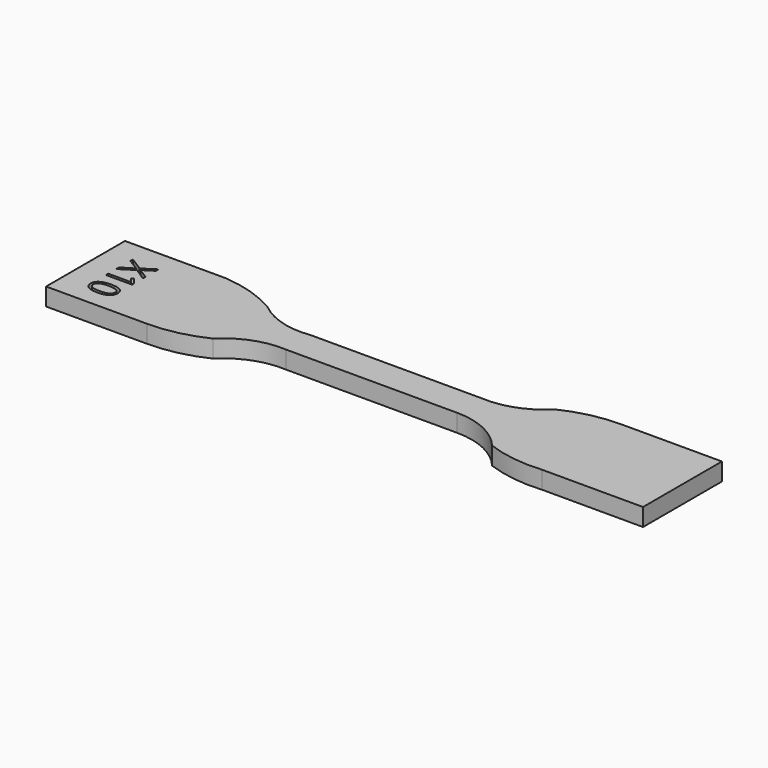
from build123d import *

# Parameters (mm, degrees)
F1_DEPTH     = 3.4
F2_TEXT_SIZE = 7.0564552314
F3_DEPTH     = 1


# Not quite as in the source:
# - Text() gives the source's letters only with a copy of the font that has no kerning and outlines rounded to 1/6400 em; it was checked with that copy


with BuildPart() as f1:
    # F0 (on Top) → F1 (new body)
    with BuildSketch(Plane.XY):
        with BuildLine():
            Line((-14.4320548165, 19.7811394548), (-33.8720548165, 19.7811394548))
            Line((-33.8720548165, 19.7811394548), (-33.8720548165, 0.7811394548))
            Line((-33.8720548165, 0.7811394548), (-14.4320548165, 0.7811394548))
            ThreePointArc((-14.4320548165, 0.7811394548), (-8.9053122052, 1.3996892086), (-3.6520548165, 3.2247301661))
            ThreePointArc((-3.6520548165, 3.2247301661), (1.3014698263, 6.4128780055), (7.1279451835, 7.2811394548))
            Line((7.1279451835, 7.2811394548), (40.1279451835, 7.2811394548))
            ThreePointArc((40.1279451835, 7.2811394548), (46.0837574042, 5.9511158081), (50.9079451835, 2.2137538538))
            ThreePointArc((50.9079451835, 2.2137538538), (56.2191047011, 0.9041953221), (61.6879451835, 0.7811394548))
            Line((61.6879451835, 0.7811394548), (81.1279451835, 0.7811394548))
            Line((81.1279451835, 0.7811394548), (81.1279451835, 19.7811394548))
            Line((81.1279451835, 19.7811394548), (61.6879451835, 19.7811394548))
            ThreePointArc((61.6879451835, 19.7811394548), (56.1612025723, 19.162589701), (50.9079451835, 17.3375487435))
            ThreePointArc((50.9079451835, 17.3375487435), (45.9544205407, 14.1494009041), (40.1279451835, 13.2811394548))
            Line((40.1279451835, 13.2811394548), (7.1279451835, 13.2811394548))
            ThreePointArc((7.1279451835, 13.2811394548), (1.4167452884, 13.6925537245), (-3.6520548165, 16.3560723447))
            ThreePointArc((-3.6520548165, 16.3560723447), (-8.8458057958, 18.686276846), (-14.4320548165, 19.7811394548))
        make_face()
    extrude(amount=F1_DEPTH)

    # F2 (on face) → F3 (cut)
    with BuildSketch(Plane.XY.offset(3.4)):
        with Locations(Location((-29.1824135929, 15.8650862949), (0, 0, -90))):
            Text('X10', F2_TEXT_SIZE, font='Open Sans', text_align=(TextAlign.LEFT, TextAlign.BOTTOM))
    extrude(amount=-F3_DEPTH, mode=Mode.SUBTRACT)


solid = f1.part
